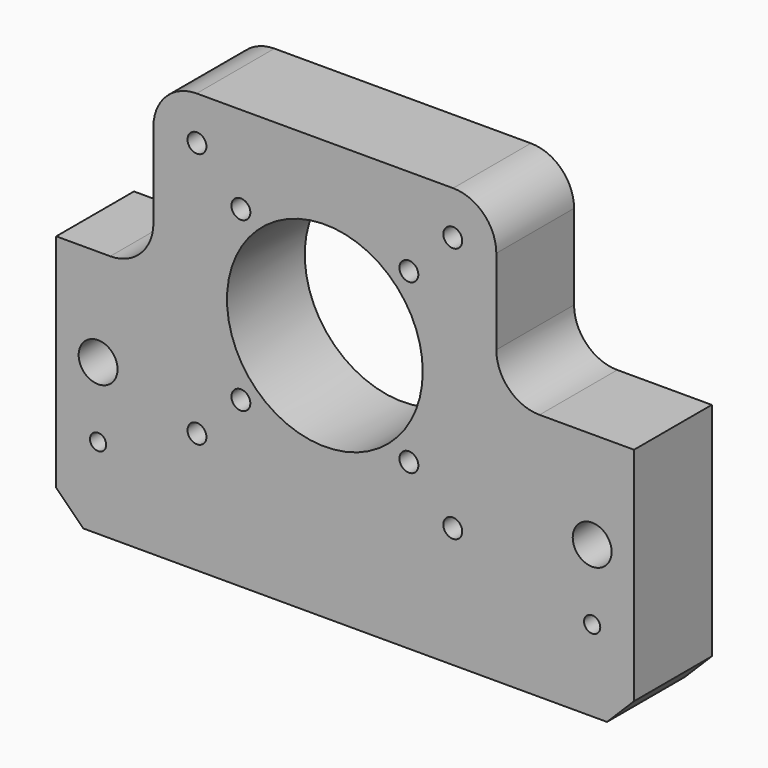
from build123d import *

# Parameters (mm, degrees)
F0_R           = 1.75
F0_R_2         = 1.5
F1_DEPTH       = 18
F2_SIZE        = 5
F3_R           = 8
F4_D           = 7.2
F4_DEPTH       = 35
F4_CBORE_D     = 11
F4_CBORE_DEPTH = 6
F4_TIP         = 2.1630982285


# Not quite as in the source:
# - a feature names something its author has since deleted; it is built from what else it names


with BuildPart() as f1:
    # F0 (on Front) → F1 (new body)
    with BuildSketch(Plane.XZ):
        with BuildLine():
            ThreePointArc((-18.125, 0), (0, 18.125), (18.125, 0))
            Line((18.125, 0), (31.75, 0))
            Line((31.75, 0), (31.75, 31.75))
            Line((31.75, 31.75), (-31.75, 31.75))
            Line((-31.75, 31.75), (-31.75, 0))
            Line((-31.75, 0), (-18.125, 0))
        make_face()
        with Locations((-23.6880771697, 23.6880771697)):
            Circle(F0_R, mode=Mode.SUBTRACT)
        with Locations((-15.5563491861, 15.5563491861)):
            Circle(F0_R, mode=Mode.SUBTRACT)
        with Locations((15.5563491861, 15.5563491861)):
            Circle(F0_R, mode=Mode.SUBTRACT)
        with Locations((23.6880771697, 23.6880771697)):
            Circle(F0_R, mode=Mode.SUBTRACT)
        with BuildLine():
            Line((31.75, 0), (18.125, 0))
            ThreePointArc((18.125, 0), (0, -18.125), (-18.125, 0))
            Line((-18.125, 0), (-31.75, 0))
            Line((-31.75, 0), (-31.75, -31.75))
            Line((-31.75, -31.75), (31.75, -31.75))
            Line((31.75, -31.75), (31.75, 0))
        make_face()
        with Locations((-23.6880771697, -23.6880771697)):
            Circle(F0_R, mode=Mode.SUBTRACT)
        with Locations((-15.5563491861, -15.5563491861)):
            Circle(F0_R, mode=Mode.SUBTRACT)
        with Locations((23.6880771697, -23.6880771697)):
            Circle(F0_R, mode=Mode.SUBTRACT)
        with Locations((15.5563491861, -15.5563491861)):
            Circle(F0_R, mode=Mode.SUBTRACT)
        Polygon((57.25, 0), (31.75, 0), (31.75, -31.75), (-31.75, -31.75), (-31.75, 0), (-49.75, 0), (-49.75, -46), (57.25, -46), align=None)
        with Locations((-42, -31)):
            Circle(F0_R_2, mode=Mode.SUBTRACT)
        with Locations((49.5, -31)):
            Circle(F0_R_2, mode=Mode.SUBTRACT)
    extrude(amount=F1_DEPTH)

    # F2
    f2_edges = [f1.edges().sort_by_distance(p)[0] for p in [
        (-49.75, -9, -46),
        (57.25, -9, -46),
    ]]
    chamfer(f2_edges, length=F2_SIZE)

    # F3
    f3_edges = [f1.edges().sort_by_distance(p)[0] for p in [
        (-31.75, -9, 0),
        (-31.75, -9, 31.75),
        (31.75, -9, 31.75),
        (31.75, -9, 0),
    ]]
    fillet(f3_edges, radius=F3_R)

    # F4
    with Locations(Plane(origin=(0, 0, 0), x_dir=(1, 0, 0), z_dir=(0, 1, 0))):
        with Locations((49.5, 18), (-42, 18)):
            CounterBoreHole(F4_D / 2, F4_CBORE_D / 2, F4_CBORE_DEPTH, depth=F4_DEPTH)
            with Locations((0, 0, -(F4_DEPTH + F4_TIP / 2))):  # 118° drill point
                Cone(0, F4_D / 2, F4_TIP, mode=Mode.SUBTRACT)


solid = f1.part
